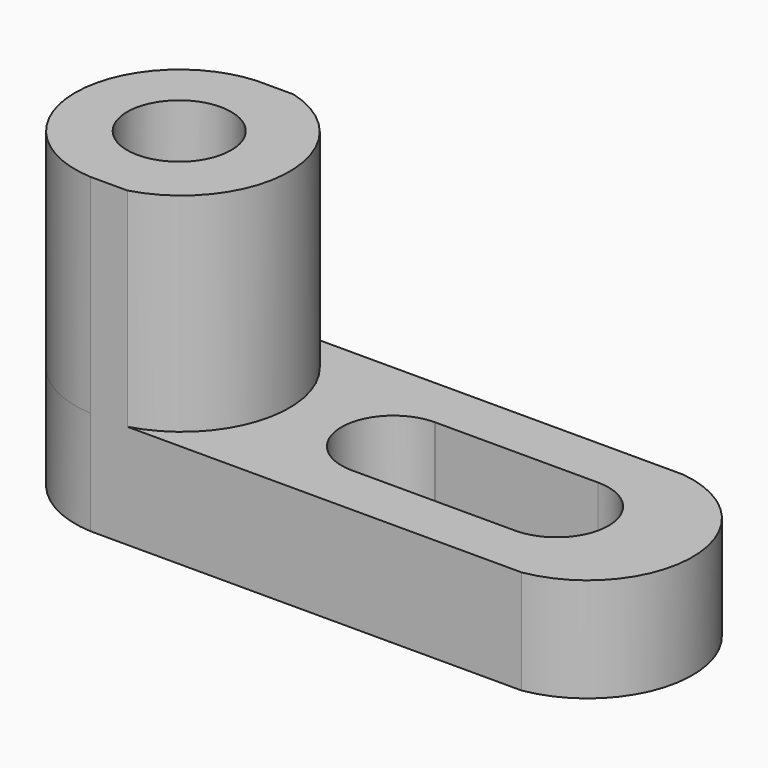
from build123d import *

# Parameters (mm, degrees)
F0_W      = 76.2
F0_H      = 12.7
F1_DEPTH  = 25.4
F3_DEPTH  = 25.4
F4_R      = 6.35
F5_DEPTH  = 50.8
F7_DEPTH  = 25.4
F8_R      = 6.35
F10_DEPTH = 25.4
F12_DEPTH = 25.4
F13_DEPTH = 25.4


# Not quite as in the source:
# - ends of sketch curves that miss each other by under 0.0002 mm in the source are joined


with BuildPart() as f1:
    # F0 (on Front) → F1 (new body)
    with BuildSketch(Plane.XZ):
        with Locations((38.1, 6.35)):
            Rectangle(F0_W, F0_H)
    extrude(amount=F1_DEPTH)

    # F2 (on face) → F3 (cut)
    with BuildSketch(Plane.XY.offset(12.7)):
        with BuildLine():
            ThreePointArc((64.0390142798, 0), (75.4038787349, -12.4300591202), (64.6592453122, -25.4))
            Line((64.6592453122, -25.4), (76.2, -25.4))
            Line((76.2, -25.4), (76.2, 0))
            Line((76.2, 0), (64.0390142798, 0))
        make_face()
    extrude(amount=-F3_DEPTH, mode=Mode.SUBTRACT)

    # F4 (on face) → F5 (cut)
    with BuildSketch(Plane.XY.offset(12.7)):
        with BuildLine():
            ThreePointArc((12.0300554493, -25.4), (3.4859185716, -21.4578724796), (-1.23091e-05, -12.717681963))
            Line((-1.23091e-05, -12.717681963), (0, -25.4))
            Line((0, -25.4), (12.0300554493, -25.4))
        make_face()
        with Locations((12.6999876909, -12.717681963)):
            Circle(F4_R)
    extrude(amount=-F5_DEPTH, mode=Mode.SUBTRACT)

    # F6 (on face) → F7 (cut)
    with BuildSketch(Plane.XY.offset(12.7)):
        with BuildLine():
            ThreePointArc((0, -12.735363926), (3.4749459355, -3.9839181288), (12.0067364357, 0))
            Line((12.0067364357, 0), (0, 0))
            Line((0, 0), (0, -12.735363926))
        make_face()
    extrude(amount=-F7_DEPTH, mode=Mode.SUBTRACT)

    # F8 (on face) → F10 (join)
    with BuildSketch(Plane.XY.offset(12.7)):
        with BuildLine():
            Line((12.0300554493, -25.4), (16.5153164417, -25.4))
            ThreePointArc((16.5153164417, -25.4), (26.1494098267, -12.7), (16.5153164417, 0))
            Line((16.5153164417, 0), (12.0067364357, 0))
            ThreePointArc((12.0067364357, 0), (3.4749459355, -3.9839181288), (0, -12.735363926))
            ThreePointArc((0, -12.735363926), (3.4920052044, -21.4642846479), (12.0300554493, -25.4))
        make_face()
        with Locations((12.6999876909, -12.717681963)):
            Circle(F8_R, mode=Mode.SUBTRACT)
    extrude(amount=F10_DEPTH)

    # F11 (on face) → F12 (cut)
    with BuildSketch(Plane.XY.offset(12.7)):
        with BuildLine():
            Line((39.0294717837, -19.0474465489), (58.5869699212, -19.0474465489))
            ThreePointArc((58.5869699212, -19.0474465489), (52.4176695499, -12.6100109835), (58.7669298396, -6.3500000008))
            Line((58.7669298396, -6.3500000008), (38.9130622506, -6.3503190341))
            ThreePointArc((38.9130622506, -6.3503190341), (43.361986302, -8.2324331506), (45.1994098267, -12.7))
            ThreePointArc((45.1994098267, -12.7), (43.4027543902, -17.126008731), (39.0294717837, -19.0474465489))
        make_face()
        with BuildLine():
            Line((38.6693478697, -19.0474465489), (39.0294717837, -19.0474465489))
            ThreePointArc((39.0294717837, -19.0474465489), (43.4027543902, -17.126008731), (45.1994098267, -12.7))
            ThreePointArc((45.1994098267, -12.7), (43.361986302, -8.2324331506), (38.9130622506, -6.3503190341))
            ThreePointArc((38.9130622506, -6.3503190341), (38.8493077881, -6.3500000008), (38.7855533359, -6.350321083))
            ThreePointArc((38.7855533359, -6.350321083), (32.4996757514, -12.6418865466), (38.6693478697, -19.0474465489))
        make_face()
    extrude(amount=-F12_DEPTH, mode=Mode.SUBTRACT)

    # F9 (on face) → F13 (cut)
    with BuildSketch(Plane.XY.offset(12.7)):
        with BuildLine():
            Line((38.9130622506, -6.3503190341), (38.7855533359, -6.350321083))
            ThreePointArc((38.7855533359, -6.350321083), (32.4994908094, -12.7320698283), (38.8496921889, -19.0499999937))
            ThreePointArc((38.8496921889, -19.0499999937), (43.3396377163, -17.1900282293), (45.1994098267, -12.7))
            ThreePointArc((45.1994098267, -12.7), (43.361986302, -8.2324331506), (38.9130622506, -6.3503190341))
        make_face()
        with BuildLine():
            ThreePointArc((45.1994098267, -12.7), (43.3396377163, -17.1900282293), (38.8496921889, -19.0499999937))
            Line((38.8496921889, -19.0499999937), (58.6612614637, -19.0491190428))
            ThreePointArc((58.6612614637, -19.0491190428), (52.4172516966, -12.6471639759), (58.7669298396, -6.3500000008))
            Line((58.7669298396, -6.3500000008), (38.9130622506, -6.3503190341))
            ThreePointArc((38.9130622506, -6.3503190341), (43.361986302, -8.2324331506), (45.1994098267, -12.7))
        make_face()
        with BuildLine():
            Line((58.8733669384, -19.0491096112), (58.6612614637, -19.0491190428))
            ThreePointArc((58.6612614637, -19.0491190428), (58.7673142404, -19.0499999937), (58.8733669384, -19.0491096112))
        make_face()
        with BuildLine():
            ThreePointArc((58.7669298396, -6.3500000008), (52.4172516966, -12.6471639759), (58.6612614637, -19.0491190428))
            Line((58.6612614637, -19.0491190428), (58.8733669384, -19.0491096112))
            ThreePointArc((58.8733669384, -19.0491096112), (63.294598975, -17.1523742188), (65.1170318782, -12.7))
            ThreePointArc((65.1170318782, -12.7), (63.2571238625, -8.2098358635), (58.7669298396, -6.3500000008))
        make_face()
    extrude(amount=-F13_DEPTH, mode=Mode.SUBTRACT)


solid = f1.part
